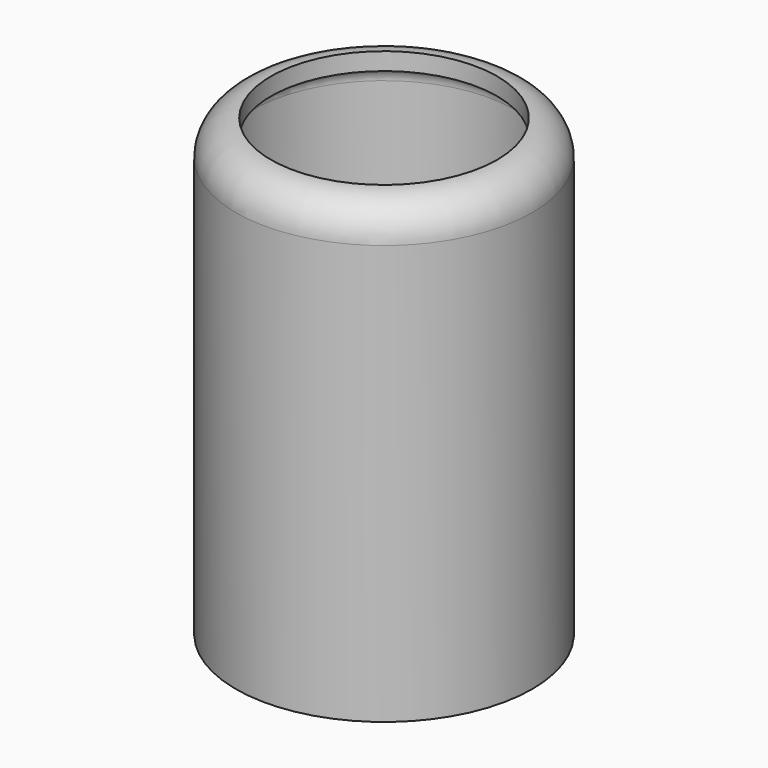
from build123d import *

# Parameters (mm, degrees)
F0_R     = 21.4542850261
F1_DEPTH = 65.786
F2_R     = 5.08
F3_T     = -2.54


# Not quite as in the source:
# - a shell that OpenCascade refuses in one call is made with other operations: the cavity is built on its own and cut out


with BuildPart() as f1:
    # F0 (on Top) → F1 (new body)
    with BuildSketch(Plane.XY):
        with Locations((-44.2928858101, 29.3457191437)):
            Circle(F0_R)
    extrude(amount=F1_DEPTH)

    # F2
    f2_edges = [f1.edges().sort_by_distance(p)[0] for p in [
        (-65.747171, 29.345719, 65.786),
    ]]
    fillet(f2_edges, radius=F2_R)

    # F3: a shell. OpenCascade refuses it in one call, so the cavity is built on its own and cut out:
    # the body offset inwards by the wall thickness, plus a prism from it out through each open face.
    f3_core = offset(f1.part, amount=F3_T, mode=Mode.PRIVATE)
    f3_exits = [f3_core.faces().sort_by_distance(p)[0] for p in [
        (-44.292886, 29.345719, 63.246),
    ]]
    add(f3_core, mode=Mode.SUBTRACT)
    extrude(f3_exits, amount=-F3_T, mode=Mode.SUBTRACT)


solid = f1.part
